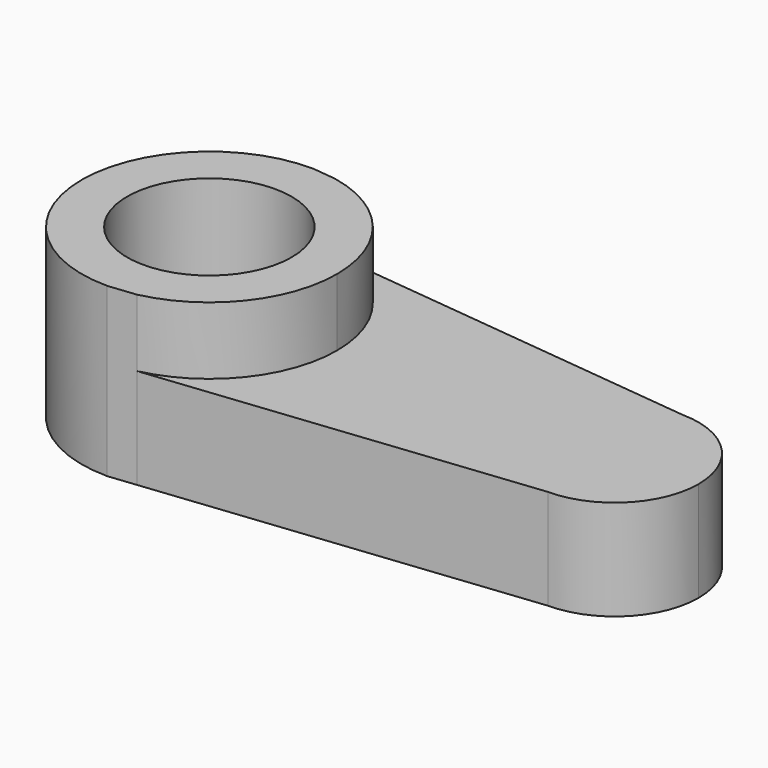
from build123d import *

# Parameters (mm, degrees)
F1_DEPTH = 3.29
F0_R     = 2.7
F2_DEPTH = 5.5


with BuildPart() as f1:
    # F0 (on Top) → F1 (new body)
    with BuildSketch(Plane.XY):
        with BuildLine():
            Line((18.7677565455, 12.2794405385), (6.2668947811, 13.6353748107))
            ThreePointArc((6.2668947811, 13.6353748107), (8.675985762, 12.1804513231), (9.621155417, 9.5295691997))
            ThreePointArc((9.621155417, 9.5295691997), (8.6954252879, 6.9026618527), (6.3272927871, 5.4365217026))
            Line((6.3272927871, 5.4365217026), (18.741155417, 6.7795691997))
            ThreePointArc((18.741155417, 6.7795691997), (15.9911875825, 9.5428699196), (18.7677565455, 12.2794405385))
        make_face()
        with BuildLine():
            ThreePointArc((21.491155417, 9.5295691997), (20.69508135, 11.4646850744), (18.7677565455, 12.2794405385))
            ThreePointArc((18.7677565455, 12.2794405385), (15.9911875825, 9.5428699196), (18.741155417, 6.7795691997))
            ThreePointArc((18.741155417, 6.7795691997), (20.6856990652, 7.5850255515), (21.491155417, 9.5295691997))
        make_face()
    extrude(amount=F1_DEPTH)

    # F0 (on Top) → F2 (join)
    with BuildSketch(Plane.XY):
        with BuildLine():
            Line((6.2668947811, 13.6353748107), (5.4951863181, 13.7190799162))
            ThreePointArc((5.4951863181, 13.7190799162), (1.2412777396, 9.561585585), (5.431155417, 5.3395691997))
            Line((5.431155417, 5.3395691997), (6.3272927871, 5.4365217026))
            ThreePointArc((6.3272927871, 5.4365217026), (8.6954252879, 6.9026618527), (9.621155417, 9.5295691997))
            ThreePointArc((9.621155417, 9.5295691997), (8.675985762, 12.1804513231), (6.2668947811, 13.6353748107))
        make_face()
        with Locations((5.431155417, 9.5295691997)):
            Circle(F0_R, mode=Mode.SUBTRACT)
    extrude(amount=F2_DEPTH)


solid = f1.part
